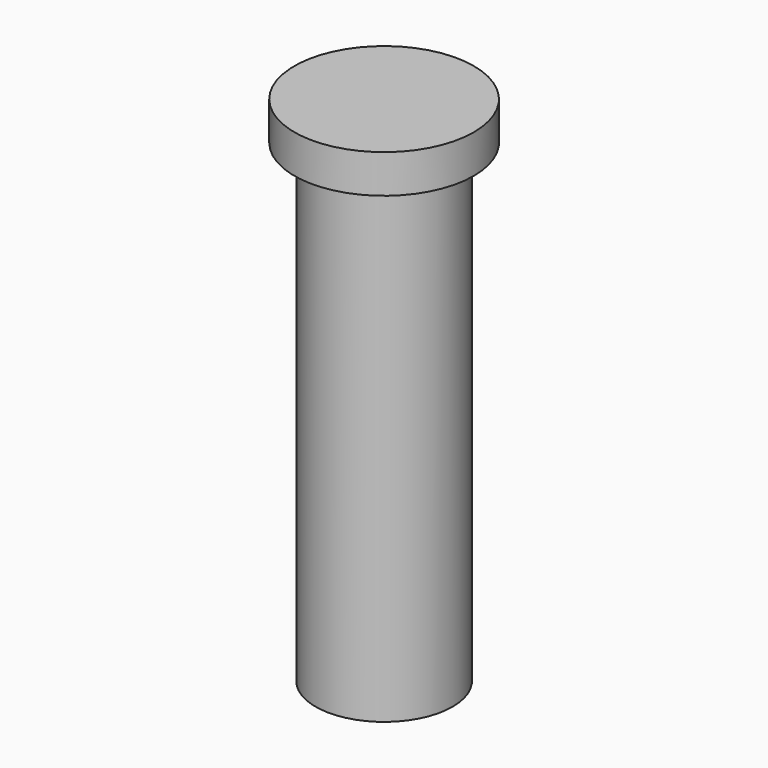
from build123d import *


# Not quite as in the source:
# - a feature names something its author has since deleted; it is built from what else it names


with BuildPart() as f1:
    # F0 (on Front) → F1 (revolve)
    with BuildSketch(Plane.XZ):
        Polygon((0, 40), (0, 0), (5.35, 0), (5.35, 37), (7, 37), (7, 40), align=None)
    revolve(axis=Axis((0, 0, 23.8549038768), (0, 0, 1)))


solid = f1.part
